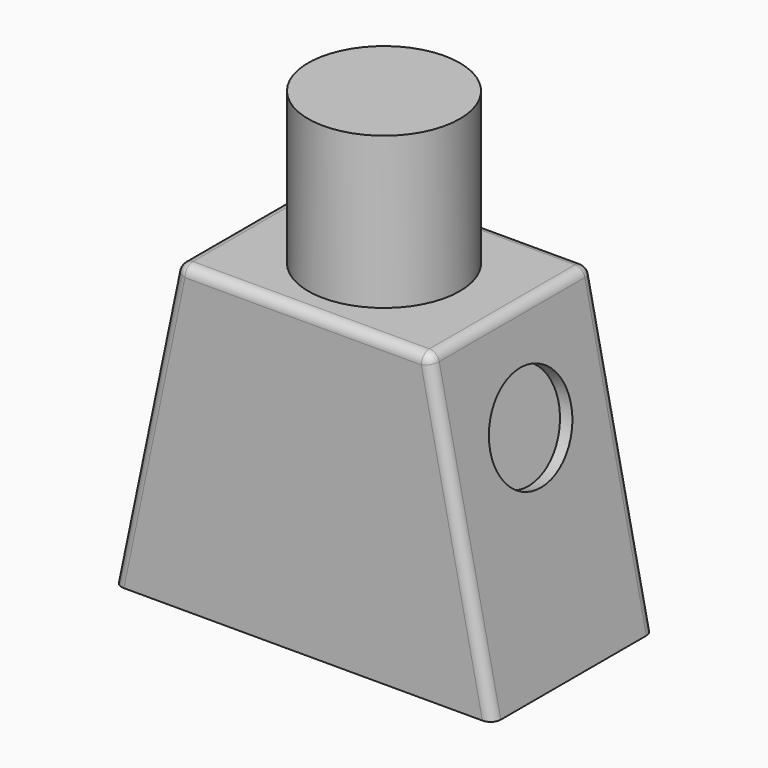
from build123d import *

# Parameters (mm, degrees)
F1_DEPTH = 8
F2_T     = -0.5
F3_W     = 13.9785291107
F3_H     = 7
F4_DEPTH = 0.5
F5_R     = 0.4
F6_R     = 2
F7_DEPTH = 1
F8_R     = 3
F9_DEPTH = 6


# Not quite as in the source:
# - a pattern or mirror of a feature is missing from the dataset's text; its kind, count and spacing are read off the source's solid


with BuildPart() as f1:
    # F0 (on Front) → F1 (new body)
    with BuildSketch(Plane.XZ):
        Polygon((-7.5, 0), (0, 0), (7.5, 0), (5, 12), (0, 12), (-5, 12), align=None)
    extrude(amount=F1_DEPTH)

    # F2
    f2_openings = [f1.faces().sort_by_distance(p)[0] for p in [
        (0, -4, 0),
    ]]
    offset(amount=F2_T, openings=f2_openings)

    # F3 (on face) → F4 (cut)
    with BuildSketch(Plane(origin=(0, 0, 0), x_dir=(1, 0, 0), z_dir=(0, 0, -1))):
        with Locations((0, 4)):
            Rectangle(F3_W, F3_H)
    extrude(amount=-F4_DEPTH, mode=Mode.SUBTRACT)

    # F5
    f5_edges = [f1.edges().sort_by_distance(p)[0] for p in [
        (6.25, -8, 6),
        (5, -4, 12),
        (0, -8, 12),
        (6.25, 0, 6),
        (0, 0, 12),
        (-6.25, 0, 6),
        (-5, -4, 12),
        (-6.25, -8, 6),
    ]]
    fillet(f5_edges, radius=F5_R)

    # F6 (on face) → F7 (cut)
    with BuildSketch(Plane(origin=(-7.1880199667, 0, 1.4975041597), x_dir=(0, -1, 0), z_dir=(-0.9789804197, 0, 0.2039542541))):
        with Locations((4, 6.8027387439)):
            Circle(F6_R)
    f7 = extrude(amount=-F7_DEPTH, mode=Mode.SUBTRACT)

    # F7_copies: F7 across plane
    add(f7.mirror(Plane(origin=(0, 0, 0), x_dir=(0, 0, 1), z_dir=(1, 0, 0))), mode=Mode.SUBTRACT)

    # F8 (on face) → F9 (join)
    with BuildSketch(Plane.XY.offset(12)):
        with Locations((0, -4)):
            Circle(F8_R)
    extrude(amount=F9_DEPTH)


solid = f1.part
